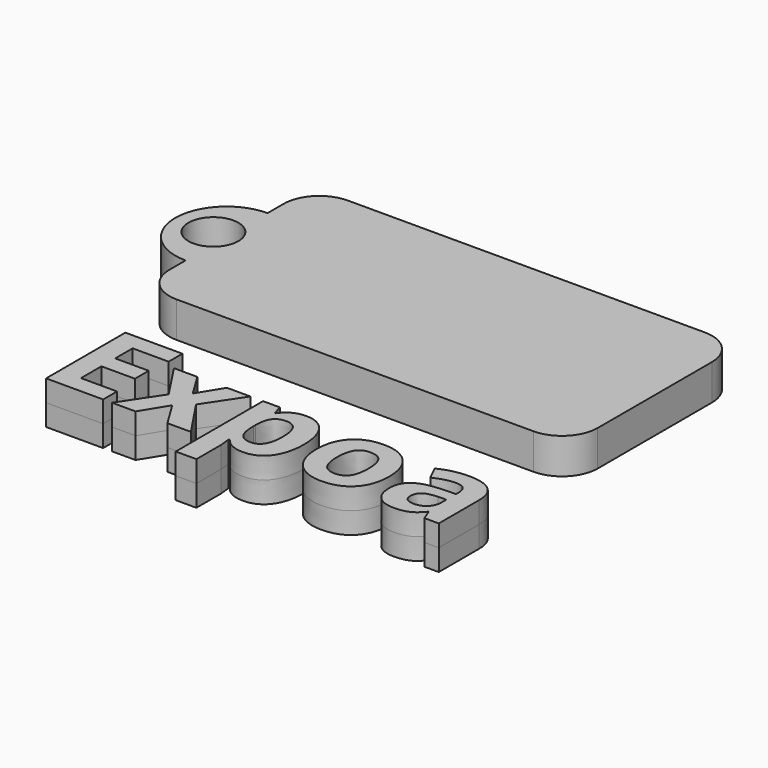
from build123d import *

# Parameters (mm, degrees)
F1_DEPTH     = 5
F2_R         = 5
F3_DEPTH     = 5
F4_R         = 1.786161763
F5_DEPTH     = 25
F6_TEXT_SIZE = 19.4444444444
F7_DEPTH     = 3
F4_R_2       = 3.5
F8_DEPTH     = 25
F9_DEPTH     = 3


# Not quite as in the source:
# - Text() gives the source's letters only with a copy of the font that has no kerning and outlines rounded to 1/6400 em; it was checked with that copy


with BuildPart() as f1:
    # F0 (on Top) → F1 (new body)
    with BuildSketch(Plane.XY):
        with BuildLine():
            Line((-30, -15), (30, -15))
            Line((30, -15), (30, 15))
            Line((30, 15), (-30, 15))
            Line((-30, 15), (-30, 7.1789468883))
            ThreePointArc((-30, 7.1789468883), (-24.9237179735, 5.0762820265), (-22.8210531117, 0))
            ThreePointArc((-22.8210531117, 0), (-24.9237179735, -5.0762820265), (-30, -7.1789468883))
            Line((-30, -7.1789468883), (-30, -15))
        make_face()
    extrude(amount=F1_DEPTH)

    # F2
    f2_edges = [f1.edges().sort_by_distance(p)[0] for p in [
        (-30, -15, 2.5),
        (30, -15, 2.5),
        (30, 15, 2.5),
        (-30, 15, 2.5),
    ]]
    fillet(f2_edges, radius=F2_R)

    # F0 (on Top) → F3 (join)
    with BuildSketch(Plane.XY):
        with BuildLine():
            Line((-30, 7.1789468883), (-30, -7.1789468883))
            ThreePointArc((-30, -7.1789468883), (-24.9237179735, -5.0762820265), (-22.8210531117, 0))
            ThreePointArc((-22.8210531117, 0), (-24.9237179735, 5.0762820265), (-30, 7.1789468883))
        make_face()
        with BuildLine():
            ThreePointArc((-30, 7.1789468883), (-37.1789468883, 0), (-30, -7.1789468883))
            Line((-30, -7.1789468883), (-30, 7.1789468883))
        make_face()
    extrude(amount=F3_DEPTH)

    # F4 (on face) → F5 (cut)
    with BuildSketch(Plane.XY.offset(5)):
        with Locations((-31.8425856531, 0)):
            Circle(F4_R)
    extrude(amount=-F5_DEPTH, mode=Mode.SUBTRACT)

    # F4 (on face) → F8 (cut)
    with BuildSketch(Plane.XY.offset(5)):
        with Locations((-31.8425856531, 0)):
            Circle(F4_R_2)
        with Locations((-31.8425856531, 0)):
            Circle(F4_R, mode=Mode.SUBTRACT)
        with Locations((-31.8425856531, 0)):
            Circle(F4_R)
    extrude(amount=-F8_DEPTH, mode=Mode.SUBTRACT)


with BuildPart() as f7:
    # F6 (on Top) → F7 (new body)
    with BuildSketch(Plane.XY):
        with Locations((-28.6098690341, -35.5220428379)):
            Text('Expoa', F6_TEXT_SIZE, font='Open Sans', font_style=FontStyle.BOLD, text_align=(TextAlign.LEFT, TextAlign.BOTTOM))
    extrude(amount=-F7_DEPTH)


with BuildPart() as f9:
    # F6 (on Top) → F9 (new body)
    with BuildSketch(Plane.XY):
        with Locations((-28.6098690341, -35.5220428379)):
            Text('Expoa', F6_TEXT_SIZE, font='Open Sans', font_style=FontStyle.BOLD, text_align=(TextAlign.LEFT, TextAlign.BOTTOM))
    extrude(amount=F9_DEPTH)


solid = Compound([f1.part, f7.part, f9.part])
